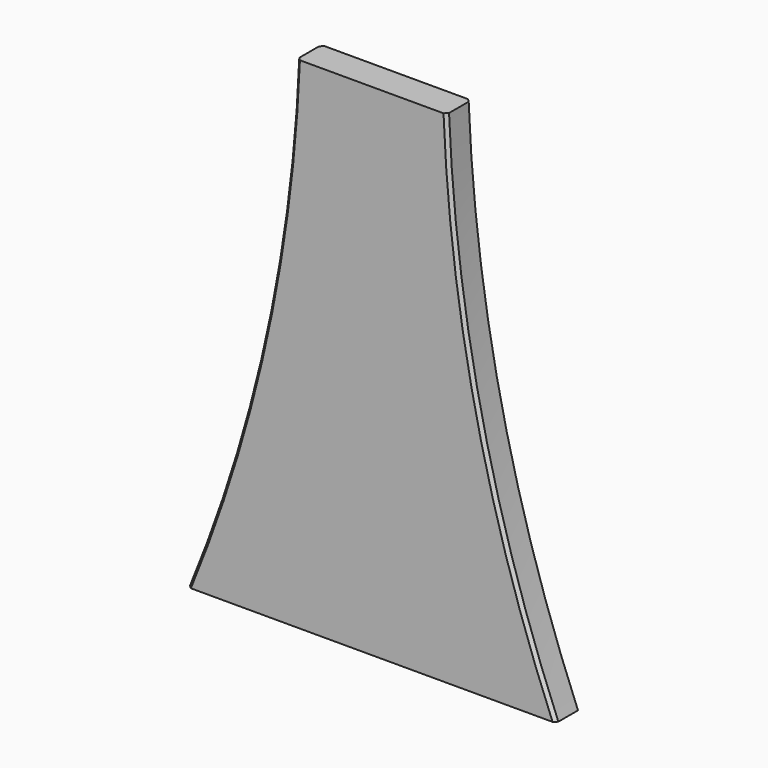
from build123d import *

# Parameters (mm, degrees)
F1_DEPTH = 5
F2_SIZE  = 0.5


# Not quite as in the source:
# - ends of sketch curves that miss each other by under 0.0002 mm in the source are joined


with BuildPart() as f1:
    # F0 (on Front) → F1 (new body)
    with BuildSketch(Plane.XZ):
        with BuildLine():
            Line((12.196068, 40.75), (-12.196068, 40.75))
            ThreePointArc((-12.196068, 40.75), (-17.5303965634, -0.7793616591), (-30, -40.75))
            Line((-30, -40.75), (30, -40.75))
            ThreePointArc((30, -40.75), (17.5303965634, -0.7793616591), (12.196068, 40.75))
        make_face()
    extrude(amount=F1_DEPTH)

    # F2
    f2_edges = [f1.edges().sort_by_distance(p)[0] for p in [
        (-17.530397, 0, -0.779362),
        (-17.530397, -5, -0.779362),
        (17.530397, -5, -0.779362),
        (17.530397, 0, -0.779362),
    ]]
    chamfer(f2_edges, length=F2_SIZE)


solid = f1.part
